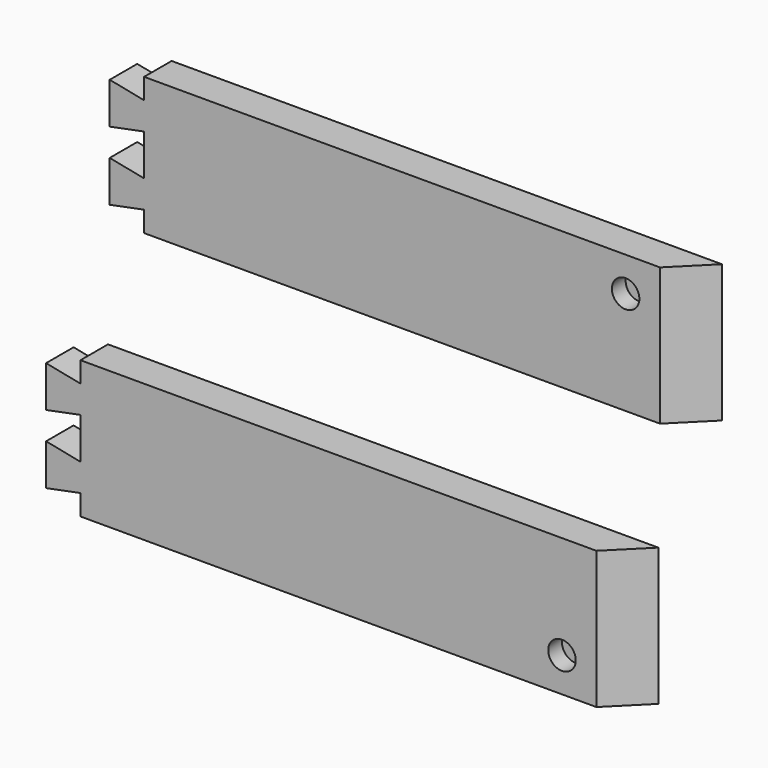
from build123d import *

# Parameters (mm, degrees)
F1_DEPTH = 10
F2_SIZE  = 9.99999
F3_SIZE  = 9.99999
F4_R     = 4
F5_DEPTH = 5
F6_R     = 4
F7_DEPTH = 5


# Not quite as in the source:
# - a fillet or chamfer is up to 0.001 mm smaller than in the source, because OpenCascade refuses the exact size


with BuildPart() as f1:
    # F0 (on Front) → F1 (new body)
    with BuildSketch(Plane.XZ):
        Polygon((10, 6), (10, 0), (170, 0), (170, 40), (10, 40), (10, 34), (0, 36), (0, 24), (10, 26), (10, 14), (0, 16), (0, 4), align=None)
    extrude(amount=F1_DEPTH)

    # F2 (size 10 in the source; OpenCascade refuses exactly that, so slightly less here)
    f2_edges = [f1.edges().sort_by_distance(p)[0] for p in [
        (170, -10, 20),
    ]]
    chamfer(f2_edges, length=F2_SIZE)

    # F4 (on face) → F5 (cut)
    with BuildSketch(Plane.XZ.offset(10)):
        with Locations((150, 30)):
            Circle(F4_R)
    extrude(amount=-F5_DEPTH, mode=Mode.SUBTRACT)


with BuildPart() as f1b:
    # F0 (on Front) → F1, piece 2 (new body)
    with BuildSketch(Plane.XZ):
        Polygon((-8.5003077292, -72.550413698), (-8.5003077292, -78.550413698), (151.4996922708, -78.550413698), (151.4996922708, -38.550413698), (-8.5003077292, -38.550413698), (-8.5003077292, -44.550413698), (-18.5003077292, -42.550413698), (-18.5003077292, -54.550413698), (-8.5003077292, -52.550413698), (-8.5003077292, -64.550413698), (-18.5003077292, -62.550413698), (-18.5003077292, -74.550413698), align=None)
    extrude(amount=F1_DEPTH)

    # F3 (size 10 in the source; OpenCascade refuses exactly that, so slightly less here)
    f3_edges = [f1b.edges().sort_by_distance(p)[0] for p in [
        (151.499692, -10, -58.550414),
    ]]
    chamfer(f3_edges, length=F3_SIZE)

    # F6 (on face) → F7 (cut)
    with BuildSketch(Plane.XZ.offset(10)):
        with Locations((131.4996922708, -68.550413698)):
            Circle(F6_R)
    extrude(amount=-F7_DEPTH, mode=Mode.SUBTRACT)


solid = Compound([f1.part, f1b.part])
